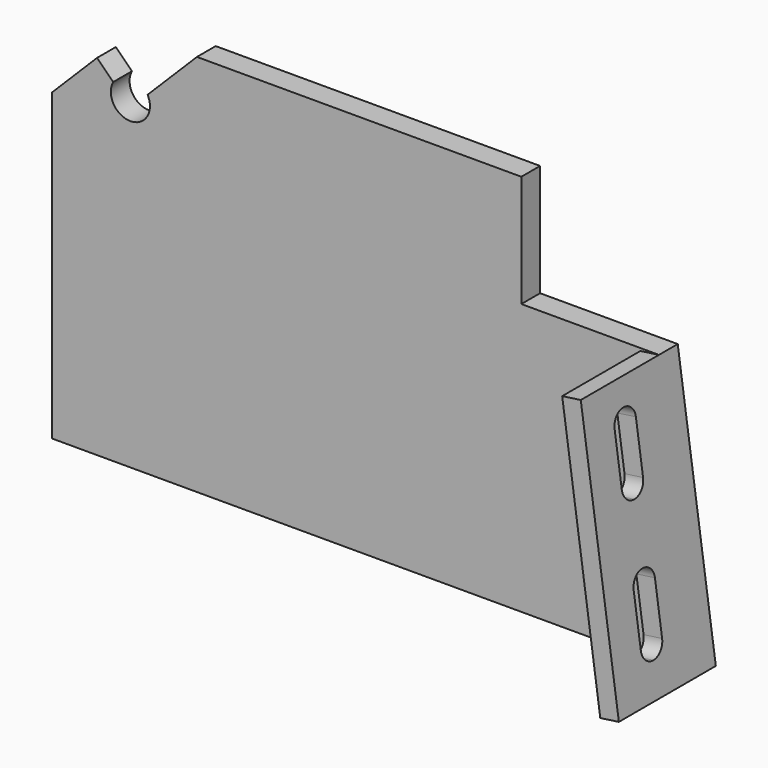
from build123d import *

# Parameters (mm, degrees)
F1_DEPTH  = 15.875
F2_W      = 4.318
F2_H      = 12.7
F3_DEPTH  = 9.175040233
F4_R      = 2.15899
F5_R      = 3.175
F6_DEPTH  = 3.81
F8_DEPTH  = 25.4
F10_DEPTH = 25.4


# Not quite as in the source:
# - a fillet or chamfer is up to 0.001 mm smaller than in the source, because OpenCascade refuses the exact size


with BuildPart() as f1:
    # F0 (on Front) → F1 (new body)
    with BuildSketch(Plane.XZ):
        Polygon((9.2045814112, -87.6168819653), (3.0183370735, -43.5994663098), (0, -44.0236659215), (6.1862443377, -88.041081577), align=None)
    extrude(amount=F1_DEPTH)

    # F2 (on face) → F3 (cut, through all)
    with BuildSketch(Plane(origin=(-6.067283434, 0, -0.8527010782), x_dir=(0, -1, 0), z_dir=(-0.9902680687, 0, -0.139173101))):
        with Locations((7.9375, -54.072730631)):
            Rectangle(F2_W, F2_H)
        with Locations((7.9375, -76.297730631)):
            Rectangle(F2_W, F2_H)
    extrude(amount=-F3_DEPTH, mode=Mode.SUBTRACT)

    # F4 (radius 2.159 in the source; OpenCascade refuses exactly that, so slightly less here)
    f4_edges = [f1.edges().sort_by_distance(p)[0] for p in [
        (2.083606, -5.7785, -47.898898),
        (5.176728, -5.7785, -69.907605),
        (5.176728, -10.0965, -69.907605),
        (2.083606, -10.0965, -47.898898),
        (3.851104, -10.0965, -60.475302),
        (6.944226, -10.0965, -82.48401),
        (6.944226, -5.7785, -82.48401),
        (3.851104, -5.7785, -60.475302),
    ]]
    fillet(f4_edges, radius=F4_R)

    # F5 (on Front) → F6 (join)
    with BuildSketch(Plane.XZ):
        Polygon((9.2045814112, -87.6168819653), (3.0183370735, -43.5994663098), (-19.3359767612, -43.5994663098), (-19.3359767612, -25.4), (-95.5359767612, -25.4), (-95.5359767612, -87.6168819653), align=None)
        with Locations((-82.8359767612, -34.925)):
            Circle(F5_R, mode=Mode.SUBTRACT)
    extrude(amount=-F6_DEPTH)

    # F7 (on Front) → F8 (cut)
    with BuildSketch(Plane.XZ):
        Polygon((-95.5359767612, -25.4), (-95.5359767612, -38.1), (-82.8359767612, -25.4), align=None)
    extrude(amount=-F8_DEPTH, mode=Mode.SUBTRACT)

    # F9 (on Front) → F10 (cut)
    with BuildSketch(Plane.XZ):
        Polygon((-70.1359767612, -23.5109585549), (-72.0250182062, -25.4), (-70.1359767612, -25.4), align=None)
        Polygon((-93.6469353161, -25.4), (-82.8359767612, -36.2109585549), (-72.0250182062, -25.4), align=None)
    extrude(amount=-F10_DEPTH, mode=Mode.SUBTRACT)


solid = f1.part
